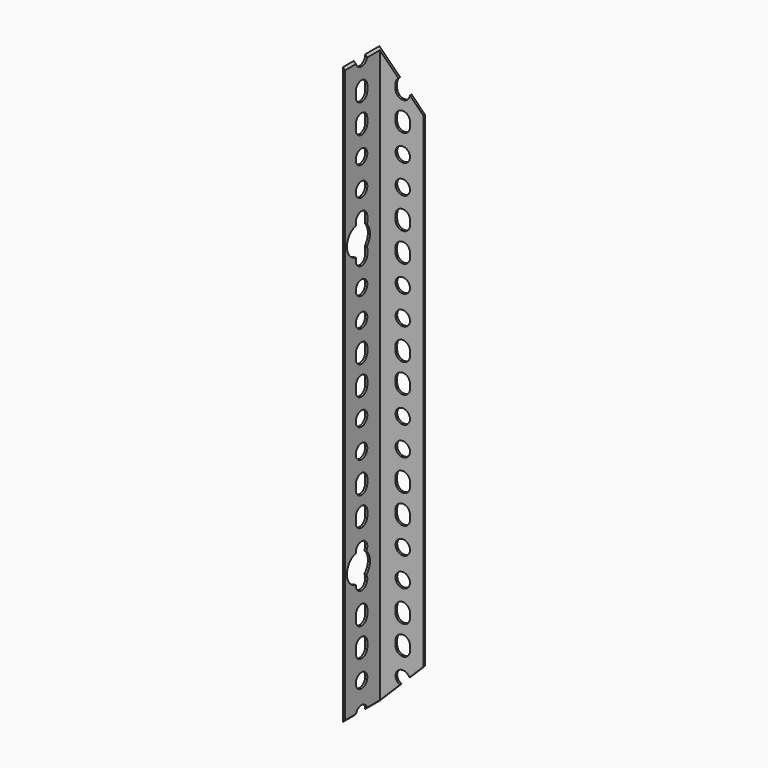
from build123d import *

# Parameters (mm, degrees)
F2_DEPTH  = 381
F3_R      = 4.7625
F5_DEPTH  = 1.3726
F4_R      = 4.7625
F6_DEPTH  = 1.3726
F8_DEPTH  = 30.1254
F10_DEPTH = 30.1254


# Not quite as in the source:
# - a variable given as a bare number and used for a length is read in inches; the dataset says mm whatever the document's units were


with BuildPart() as f2:
    # F1 (on Top) → F2 (new body)
    with BuildSketch(Plane.XY):
        Polygon((-1.3716, 1.3716), (-1.3716, -28.7528), (0, -28.7528), (0, 0), (28.7528, 0), (28.7528, 1.3716), align=None)
    extrude(amount=F2_DEPTH)

    # F3 (on face) → F5 (cut, through all)
    with BuildSketch(Plane.XZ):
        with Locations((15.1384, 19.05)):
            Circle(F3_R)
        with Locations((15.1384, 0)):
            Circle(F3_R)
        with BuildLine():
            Line((19.9009, 36.5125), (19.9009, 39.6875))
            ThreePointArc((19.9009, 39.6875), (15.1384, 44.45), (10.3759, 39.6875))
            Line((10.3759, 39.6875), (10.3759, 36.5125))
            ThreePointArc((10.3759, 36.5125), (15.1384, 31.75), (19.9009, 36.5125))
        make_face()
        with BuildLine():
            Line((19.9009, 55.5625), (19.9009, 58.7375))
            ThreePointArc((19.9009, 58.7375), (15.1384, 63.5), (10.3759, 58.7375))
            Line((10.3759, 58.7375), (10.3759, 55.5625))
            ThreePointArc((10.3759, 55.5625), (15.1384, 50.8), (19.9009, 55.5625))
        make_face()
        with BuildLine():
            Line((19.9009, 131.7625), (19.9009, 134.9375))
            ThreePointArc((19.9009, 134.9375), (15.1384, 139.7), (10.3759, 134.9375))
            Line((10.3759, 134.9375), (10.3759, 131.7625))
            ThreePointArc((10.3759, 131.7625), (15.1384, 127), (19.9009, 131.7625))
        make_face()
        with Locations((15.1384, 95.25)):
            Circle(F3_R)
        with Locations((15.1384, 76.2)):
            Circle(F3_R)
        with BuildLine():
            Line((19.9009, 112.7125), (19.9009, 115.8875))
            ThreePointArc((19.9009, 115.8875), (15.1384, 120.65), (10.3759, 115.8875))
            Line((10.3759, 115.8875), (10.3759, 112.7125))
            ThreePointArc((10.3759, 112.7125), (15.1384, 107.95), (19.9009, 112.7125))
        make_face()
        with BuildLine():
            Line((19.9009, 207.9625), (19.9009, 211.1375))
            ThreePointArc((19.9009, 211.1375), (15.1384, 215.9), (10.3759, 211.1375))
            Line((10.3759, 211.1375), (10.3759, 207.9625))
            ThreePointArc((10.3759, 207.9625), (15.1384, 203.2), (19.9009, 207.9625))
        make_face()
        with Locations((15.1384, 171.45)):
            Circle(F3_R)
        with Locations((15.1384, 152.4)):
            Circle(F3_R)
        with BuildLine():
            Line((19.9009, 188.9125), (19.9009, 192.0875))
            ThreePointArc((19.9009, 192.0875), (15.1384, 196.85), (10.3759, 192.0875))
            Line((10.3759, 192.0875), (10.3759, 188.9125))
            ThreePointArc((10.3759, 188.9125), (15.1384, 184.15), (19.9009, 188.9125))
        make_face()
        with BuildLine():
            Line((19.9009, 284.1625), (19.9009, 287.3375))
            ThreePointArc((19.9009, 287.3375), (15.1384, 292.1), (10.3759, 287.3375))
            Line((10.3759, 287.3375), (10.3759, 284.1625))
            ThreePointArc((10.3759, 284.1625), (15.1384, 279.4), (19.9009, 284.1625))
        make_face()
        with Locations((15.1384, 247.65)):
            Circle(F3_R)
        with Locations((15.1384, 228.6)):
            Circle(F3_R)
        with BuildLine():
            Line((19.9009, 265.1125), (19.9009, 268.2875))
            ThreePointArc((19.9009, 268.2875), (15.1384, 273.05), (10.3759, 268.2875))
            Line((10.3759, 268.2875), (10.3759, 265.1125))
            ThreePointArc((10.3759, 265.1125), (15.1384, 260.35), (19.9009, 265.1125))
        make_face()
        with BuildLine():
            Line((19.9009, 360.3625), (19.9009, 363.5375))
            ThreePointArc((19.9009, 363.5375), (15.1384, 368.3), (10.3759, 363.5375))
            Line((10.3759, 363.5375), (10.3759, 360.3625))
            ThreePointArc((10.3759, 360.3625), (15.1384, 355.6), (19.9009, 360.3625))
        make_face()
        with Locations((15.1384, 323.85)):
            Circle(F3_R)
        with Locations((15.1384, 304.8)):
            Circle(F3_R)
        with BuildLine():
            Line((19.9009, 341.3125), (19.9009, 344.4875))
            ThreePointArc((19.9009, 344.4875), (15.1384, 349.25), (10.3759, 344.4875))
            Line((10.3759, 344.4875), (10.3759, 341.3125))
            ThreePointArc((10.3759, 341.3125), (15.1384, 336.55), (19.9009, 341.3125))
        make_face()
        with BuildLine():
            Line((19.9009, 436.5625), (19.9009, 439.7375))
            ThreePointArc((19.9009, 439.7375), (15.1384, 444.5), (10.3759, 439.7375))
            Line((10.3759, 439.7375), (10.3759, 436.5625))
            ThreePointArc((10.3759, 436.5625), (15.1384, 431.8), (19.9009, 436.5625))
        make_face()
        with Locations((15.1384, 400.05)):
            Circle(F3_R)
        with Locations((15.1384, 381)):
            Circle(F3_R)
        with BuildLine():
            Line((19.9009, 417.5125), (19.9009, 420.6875))
            ThreePointArc((19.9009, 420.6875), (15.1384, 425.45), (10.3759, 420.6875))
            Line((10.3759, 420.6875), (10.3759, 417.5125))
            ThreePointArc((10.3759, 417.5125), (15.1384, 412.75), (19.9009, 417.5125))
        make_face()
        with BuildLine():
            Line((19.9009, 512.7625), (19.9009, 515.9375))
            ThreePointArc((19.9009, 515.9375), (15.1384, 520.7), (10.3759, 515.9375))
            Line((10.3759, 515.9375), (10.3759, 512.7625))
            ThreePointArc((10.3759, 512.7625), (15.1384, 508), (19.9009, 512.7625))
        make_face()
        with Locations((15.1384, 476.25)):
            Circle(F3_R)
        with Locations((15.1384, 457.2)):
            Circle(F3_R)
        with BuildLine():
            Line((19.9009, 493.7125), (19.9009, 496.8875))
            ThreePointArc((19.9009, 496.8875), (15.1384, 501.65), (10.3759, 496.8875))
            Line((10.3759, 496.8875), (10.3759, 493.7125))
            ThreePointArc((10.3759, 493.7125), (15.1384, 488.95), (19.9009, 493.7125))
        make_face()
        with BuildLine():
            Line((19.9009, 588.9625), (19.9009, 592.1375))
            ThreePointArc((19.9009, 592.1375), (15.1384, 596.9), (10.3759, 592.1375))
            Line((10.3759, 592.1375), (10.3759, 588.9625))
            ThreePointArc((10.3759, 588.9625), (15.1384, 584.2), (19.9009, 588.9625))
        make_face()
        with Locations((15.1384, 552.45)):
            Circle(F3_R)
        with Locations((15.1384, 533.4)):
            Circle(F3_R)
        with BuildLine():
            Line((19.9009, 569.9125), (19.9009, 573.0875))
            ThreePointArc((19.9009, 573.0875), (15.1384, 577.85), (10.3759, 573.0875))
            Line((10.3759, 573.0875), (10.3759, 569.9125))
            ThreePointArc((10.3759, 569.9125), (15.1384, 565.15), (19.9009, 569.9125))
        make_face()
        with BuildLine():
            Line((19.9009, 665.1625), (19.9009, 668.3375))
            ThreePointArc((19.9009, 668.3375), (15.1384, 673.1), (10.3759, 668.3375))
            Line((10.3759, 668.3375), (10.3759, 665.1625))
            ThreePointArc((10.3759, 665.1625), (15.1384, 660.4), (19.9009, 665.1625))
        make_face()
        with Locations((15.1384, 628.65)):
            Circle(F3_R)
        with Locations((15.1384, 609.6)):
            Circle(F3_R)
        with BuildLine():
            Line((19.9009, 646.1125), (19.9009, 649.2875))
            ThreePointArc((19.9009, 649.2875), (15.1384, 654.05), (10.3759, 649.2875))
            Line((10.3759, 649.2875), (10.3759, 646.1125))
            ThreePointArc((10.3759, 646.1125), (15.1384, 641.35), (19.9009, 646.1125))
        make_face()
        with BuildLine():
            Line((19.9009, 741.3625), (19.9009, 744.5375))
            ThreePointArc((19.9009, 744.5375), (15.1384, 749.3), (10.3759, 744.5375))
            Line((10.3759, 744.5375), (10.3759, 741.3625))
            ThreePointArc((10.3759, 741.3625), (15.1384, 736.6), (19.9009, 741.3625))
        make_face()
        with Locations((15.1384, 704.85)):
            Circle(F3_R)
        with Locations((15.1384, 685.8)):
            Circle(F3_R)
        with BuildLine():
            Line((19.9009, 722.3125), (19.9009, 725.4875))
            ThreePointArc((19.9009, 725.4875), (15.1384, 730.25), (10.3759, 725.4875))
            Line((10.3759, 725.4875), (10.3759, 722.3125))
            ThreePointArc((10.3759, 722.3125), (15.1384, 717.55), (19.9009, 722.3125))
        make_face()
        with BuildLine():
            Line((19.9009, 817.5625), (19.9009, 820.7375))
            ThreePointArc((19.9009, 820.7375), (15.1384, 825.5), (10.3759, 820.7375))
            Line((10.3759, 820.7375), (10.3759, 817.5625))
            ThreePointArc((10.3759, 817.5625), (15.1384, 812.8), (19.9009, 817.5625))
        make_face()
        with Locations((15.1384, 781.05)):
            Circle(F3_R)
        with Locations((15.1384, 762)):
            Circle(F3_R)
        with BuildLine():
            Line((19.9009, 798.5125), (19.9009, 801.6875))
            ThreePointArc((19.9009, 801.6875), (15.1384, 806.45), (10.3759, 801.6875))
            Line((10.3759, 801.6875), (10.3759, 798.5125))
            ThreePointArc((10.3759, 798.5125), (15.1384, 793.75), (19.9009, 798.5125))
        make_face()
        with BuildLine():
            Line((19.9009, 893.7625), (19.9009, 896.9375))
            ThreePointArc((19.9009, 896.9375), (15.1384, 901.7), (10.3759, 896.9375))
            Line((10.3759, 896.9375), (10.3759, 893.7625))
            ThreePointArc((10.3759, 893.7625), (15.1384, 889), (19.9009, 893.7625))
        make_face()
        with Locations((15.1384, 857.25)):
            Circle(F3_R)
        with Locations((15.1384, 838.2)):
            Circle(F3_R)
        with BuildLine():
            Line((19.9009, 874.7125), (19.9009, 877.8875))
            ThreePointArc((19.9009, 877.8875), (15.1384, 882.65), (10.3759, 877.8875))
            Line((10.3759, 877.8875), (10.3759, 874.7125))
            ThreePointArc((10.3759, 874.7125), (15.1384, 869.95), (19.9009, 874.7125))
        make_face()
        with BuildLine():
            Line((19.9009, 969.9625), (19.9009, 973.1375))
            ThreePointArc((19.9009, 973.1375), (15.1384, 977.9), (10.3759, 973.1375))
            Line((10.3759, 973.1375), (10.3759, 969.9625))
            ThreePointArc((10.3759, 969.9625), (15.1384, 965.2), (19.9009, 969.9625))
        make_face()
        with Locations((15.1384, 933.45)):
            Circle(F3_R)
        with Locations((15.1384, 914.4)):
            Circle(F3_R)
        with BuildLine():
            Line((19.9009, 950.9125), (19.9009, 954.0875))
            ThreePointArc((19.9009, 954.0875), (15.1384, 958.85), (10.3759, 954.0875))
            Line((10.3759, 954.0875), (10.3759, 950.9125))
            ThreePointArc((10.3759, 950.9125), (15.1384, 946.15), (19.9009, 950.9125))
        make_face()
        with BuildLine():
            Line((19.9009, 1046.1625), (19.9009, 1049.3375))
            ThreePointArc((19.9009, 1049.3375), (15.1384, 1054.1), (10.3759, 1049.3375))
            Line((10.3759, 1049.3375), (10.3759, 1046.1625))
            ThreePointArc((10.3759, 1046.1625), (15.1384, 1041.4), (19.9009, 1046.1625))
        make_face()
        with Locations((15.1384, 1009.65)):
            Circle(F3_R)
        with Locations((15.1384, 990.6)):
            Circle(F3_R)
        with BuildLine():
            Line((19.9009, 1027.1125), (19.9009, 1030.2875))
            ThreePointArc((19.9009, 1030.2875), (15.1384, 1035.05), (10.3759, 1030.2875))
            Line((10.3759, 1030.2875), (10.3759, 1027.1125))
            ThreePointArc((10.3759, 1027.1125), (15.1384, 1022.35), (19.9009, 1027.1125))
        make_face()
        with BuildLine():
            Line((19.9009, 1122.3625), (19.9009, 1125.5375))
            ThreePointArc((19.9009, 1125.5375), (15.1384, 1130.3), (10.3759, 1125.5375))
            Line((10.3759, 1125.5375), (10.3759, 1122.3625))
            ThreePointArc((10.3759, 1122.3625), (15.1384, 1117.6), (19.9009, 1122.3625))
        make_face()
        with Locations((15.1384, 1085.85)):
            Circle(F3_R)
        with Locations((15.1384, 1066.8)):
            Circle(F3_R)
        with BuildLine():
            Line((19.9009, 1103.3125), (19.9009, 1106.4875))
            ThreePointArc((19.9009, 1106.4875), (15.1384, 1111.25), (10.3759, 1106.4875))
            Line((10.3759, 1106.4875), (10.3759, 1103.3125))
            ThreePointArc((10.3759, 1103.3125), (15.1384, 1098.55), (19.9009, 1103.3125))
        make_face()
        with BuildLine():
            Line((19.9009, 1198.5625), (19.9009, 1201.7375))
            ThreePointArc((19.9009, 1201.7375), (15.1384, 1206.5), (10.3759, 1201.7375))
            Line((10.3759, 1201.7375), (10.3759, 1198.5625))
            ThreePointArc((10.3759, 1198.5625), (15.1384, 1193.8), (19.9009, 1198.5625))
        make_face()
        with Locations((15.1384, 1162.05)):
            Circle(F3_R)
        with Locations((15.1384, 1143)):
            Circle(F3_R)
        with BuildLine():
            Line((19.9009, 1179.5125), (19.9009, 1182.6875))
            ThreePointArc((19.9009, 1182.6875), (15.1384, 1187.45), (10.3759, 1182.6875))
            Line((10.3759, 1182.6875), (10.3759, 1179.5125))
            ThreePointArc((10.3759, 1179.5125), (15.1384, 1174.75), (19.9009, 1179.5125))
        make_face()
        with BuildLine():
            Line((19.9009, 1274.7625), (19.9009, 1277.9375))
            ThreePointArc((19.9009, 1277.9375), (15.1384, 1282.7), (10.3759, 1277.9375))
            Line((10.3759, 1277.9375), (10.3759, 1274.7625))
            ThreePointArc((10.3759, 1274.7625), (15.1384, 1270), (19.9009, 1274.7625))
        make_face()
        with Locations((15.1384, 1238.25)):
            Circle(F3_R)
        with Locations((15.1384, 1219.2)):
            Circle(F3_R)
        with BuildLine():
            Line((19.9009, 1255.7125), (19.9009, 1258.8875))
            ThreePointArc((19.9009, 1258.8875), (15.1384, 1263.65), (10.3759, 1258.8875))
            Line((10.3759, 1258.8875), (10.3759, 1255.7125))
            ThreePointArc((10.3759, 1255.7125), (15.1384, 1250.95), (19.9009, 1255.7125))
        make_face()
        with BuildLine():
            Line((19.9009, 1350.9625), (19.9009, 1354.1375))
            ThreePointArc((19.9009, 1354.1375), (15.1384, 1358.9), (10.3759, 1354.1375))
            Line((10.3759, 1354.1375), (10.3759, 1350.9625))
            ThreePointArc((10.3759, 1350.9625), (15.1384, 1346.2), (19.9009, 1350.9625))
        make_face()
        with Locations((15.1384, 1314.45)):
            Circle(F3_R)
        with Locations((15.1384, 1295.4)):
            Circle(F3_R)
        with BuildLine():
            Line((19.9009, 1331.9125), (19.9009, 1335.0875))
            ThreePointArc((19.9009, 1335.0875), (15.1384, 1339.85), (10.3759, 1335.0875))
            Line((10.3759, 1335.0875), (10.3759, 1331.9125))
            ThreePointArc((10.3759, 1331.9125), (15.1384, 1327.15), (19.9009, 1331.9125))
        make_face()
        with BuildLine():
            Line((19.9009, 1427.1625), (19.9009, 1430.3375))
            ThreePointArc((19.9009, 1430.3375), (15.1384, 1435.1), (10.3759, 1430.3375))
            Line((10.3759, 1430.3375), (10.3759, 1427.1625))
            ThreePointArc((10.3759, 1427.1625), (15.1384, 1422.4), (19.9009, 1427.1625))
        make_face()
        with Locations((15.1384, 1390.65)):
            Circle(F3_R)
        with Locations((15.1384, 1371.6)):
            Circle(F3_R)
        with BuildLine():
            Line((19.9009, 1408.1125), (19.9009, 1411.2875))
            ThreePointArc((19.9009, 1411.2875), (15.1384, 1416.05), (10.3759, 1411.2875))
            Line((10.3759, 1411.2875), (10.3759, 1408.1125))
            ThreePointArc((10.3759, 1408.1125), (15.1384, 1403.35), (19.9009, 1408.1125))
        make_face()
        with BuildLine():
            Line((19.9009, 1503.3625), (19.9009, 1506.5375))
            ThreePointArc((19.9009, 1506.5375), (15.1384, 1511.3), (10.3759, 1506.5375))
            Line((10.3759, 1506.5375), (10.3759, 1503.3625))
            ThreePointArc((10.3759, 1503.3625), (15.1384, 1498.6), (19.9009, 1503.3625))
        make_face()
        with Locations((15.1384, 1466.85)):
            Circle(F3_R)
        with Locations((15.1384, 1447.8)):
            Circle(F3_R)
        with BuildLine():
            Line((19.9009, 1484.3125), (19.9009, 1487.4875))
            ThreePointArc((19.9009, 1487.4875), (15.1384, 1492.25), (10.3759, 1487.4875))
            Line((10.3759, 1487.4875), (10.3759, 1484.3125))
            ThreePointArc((10.3759, 1484.3125), (15.1384, 1479.55), (19.9009, 1484.3125))
        make_face()
        with BuildLine():
            Line((19.9009, 1579.5625), (19.9009, 1582.7375))
            ThreePointArc((19.9009, 1582.7375), (15.1384, 1587.5), (10.3759, 1582.7375))
            Line((10.3759, 1582.7375), (10.3759, 1579.5625))
            ThreePointArc((10.3759, 1579.5625), (15.1384, 1574.8), (19.9009, 1579.5625))
        make_face()
        with Locations((15.1384, 1543.05)):
            Circle(F3_R)
        with Locations((15.1384, 1524)):
            Circle(F3_R)
        with BuildLine():
            Line((19.9009, 1560.5125), (19.9009, 1563.6875))
            ThreePointArc((19.9009, 1563.6875), (15.1384, 1568.45), (10.3759, 1563.6875))
            Line((10.3759, 1563.6875), (10.3759, 1560.5125))
            ThreePointArc((10.3759, 1560.5125), (15.1384, 1555.75), (19.9009, 1560.5125))
        make_face()
        with BuildLine():
            Line((19.9009, 1655.7625), (19.9009, 1658.9375))
            ThreePointArc((19.9009, 1658.9375), (15.1384, 1663.7), (10.3759, 1658.9375))
            Line((10.3759, 1658.9375), (10.3759, 1655.7625))
            ThreePointArc((10.3759, 1655.7625), (15.1384, 1651), (19.9009, 1655.7625))
        make_face()
        with Locations((15.1384, 1619.25)):
            Circle(F3_R)
        with Locations((15.1384, 1600.2)):
            Circle(F3_R)
        with BuildLine():
            Line((19.9009, 1636.7125), (19.9009, 1639.8875))
            ThreePointArc((19.9009, 1639.8875), (15.1384, 1644.65), (10.3759, 1639.8875))
            Line((10.3759, 1639.8875), (10.3759, 1636.7125))
            ThreePointArc((10.3759, 1636.7125), (15.1384, 1631.95), (19.9009, 1636.7125))
        make_face()
        with BuildLine():
            Line((19.9009, 1731.9625), (19.9009, 1735.1375))
            ThreePointArc((19.9009, 1735.1375), (15.1384, 1739.9), (10.3759, 1735.1375))
            Line((10.3759, 1735.1375), (10.3759, 1731.9625))
            ThreePointArc((10.3759, 1731.9625), (15.1384, 1727.2), (19.9009, 1731.9625))
        make_face()
        with Locations((15.1384, 1695.45)):
            Circle(F3_R)
        with Locations((15.1384, 1676.4)):
            Circle(F3_R)
        with BuildLine():
            Line((19.9009, 1712.9125), (19.9009, 1716.0875))
            ThreePointArc((19.9009, 1716.0875), (15.1384, 1720.85), (10.3759, 1716.0875))
            Line((10.3759, 1716.0875), (10.3759, 1712.9125))
            ThreePointArc((10.3759, 1712.9125), (15.1384, 1708.15), (19.9009, 1712.9125))
        make_face()
        with BuildLine():
            Line((19.9009, 1808.1625), (19.9009, 1811.3375))
            ThreePointArc((19.9009, 1811.3375), (15.1384, 1816.1), (10.3759, 1811.3375))
            Line((10.3759, 1811.3375), (10.3759, 1808.1625))
            ThreePointArc((10.3759, 1808.1625), (15.1384, 1803.4), (19.9009, 1808.1625))
        make_face()
        with Locations((15.1384, 1771.65)):
            Circle(F3_R)
        with Locations((15.1384, 1752.6)):
            Circle(F3_R)
        with BuildLine():
            Line((19.9009, 1789.1125), (19.9009, 1792.2875))
            ThreePointArc((19.9009, 1792.2875), (15.1384, 1797.05), (10.3759, 1792.2875))
            Line((10.3759, 1792.2875), (10.3759, 1789.1125))
            ThreePointArc((10.3759, 1789.1125), (15.1384, 1784.35), (19.9009, 1789.1125))
        make_face()
    extrude(amount=-F5_DEPTH, mode=Mode.SUBTRACT)

    # F4 (on face) → F6 (cut, through all)
    with BuildSketch(Plane.YZ):
        with Locations((-15.1384, 19.05)):
            Circle(F4_R)
        with Locations((-15.1384, 0)):
            Circle(F4_R)
        with BuildLine():
            Line((-10.3759, 36.5125), (-10.3759, 39.6875))
            ThreePointArc((-10.3759, 39.6875), (-15.1384, 44.45), (-19.9009, 39.6875))
            Line((-19.9009, 39.6875), (-19.9009, 36.5125))
            ThreePointArc((-19.9009, 36.5125), (-15.1384, 31.75), (-10.3759, 36.5125))
        make_face()
        with BuildLine():
            Line((-10.3759, 55.5625), (-10.3759, 58.7375))
            ThreePointArc((-10.3759, 58.7375), (-15.1384, 63.5), (-19.9009, 58.7375))
            Line((-19.9009, 58.7375), (-19.9009, 55.5625))
            ThreePointArc((-19.9009, 55.5625), (-15.1384, 50.8), (-10.3759, 55.5625))
        make_face()
        with BuildLine():
            Line((-10.3759, 131.7625), (-10.3759, 134.9375))
            ThreePointArc((-10.3759, 134.9375), (-15.1384, 139.7), (-19.9009, 134.9375))
            Line((-19.9009, 134.9375), (-19.9009, 131.7625))
            ThreePointArc((-19.9009, 131.7625), (-15.1384, 127), (-10.3759, 131.7625))
        make_face()
        with Locations((-15.1384, 95.25)):
            Circle(F4_R)
        with Locations((-15.1384, 76.2)):
            Circle(F4_R)
        with BuildLine():
            Line((-10.3759, 112.7125), (-10.3759, 115.8875))
            ThreePointArc((-10.3759, 115.8875), (-15.1384, 120.65), (-19.9009, 115.8875))
            Line((-19.9009, 115.8875), (-19.9009, 112.7125))
            ThreePointArc((-19.9009, 112.7125), (-15.1384, 107.95), (-10.3759, 112.7125))
        make_face()
        with BuildLine():
            Line((-10.3759, 207.9625), (-10.3759, 211.1375))
            ThreePointArc((-10.3759, 211.1375), (-15.1384, 215.9), (-19.9009, 211.1375))
            Line((-19.9009, 211.1375), (-19.9009, 207.9625))
            ThreePointArc((-19.9009, 207.9625), (-15.1384, 203.2), (-10.3759, 207.9625))
        make_face()
        with Locations((-15.1384, 171.45)):
            Circle(F4_R)
        with Locations((-15.1384, 152.4)):
            Circle(F4_R)
        with BuildLine():
            Line((-10.3759, 188.9125), (-10.3759, 192.0875))
            ThreePointArc((-10.3759, 192.0875), (-15.1384, 196.85), (-19.9009, 192.0875))
            Line((-19.9009, 192.0875), (-19.9009, 188.9125))
            ThreePointArc((-19.9009, 188.9125), (-15.1384, 184.15), (-10.3759, 188.9125))
        make_face()
        with BuildLine():
            Line((-10.3759, 284.1625), (-10.3759, 287.3375))
            ThreePointArc((-10.3759, 287.3375), (-15.1384, 292.1), (-19.9009, 287.3375))
            Line((-19.9009, 287.3375), (-19.9009, 284.1625))
            ThreePointArc((-19.9009, 284.1625), (-15.1384, 279.4), (-10.3759, 284.1625))
        make_face()
        with Locations((-15.1384, 247.65)):
            Circle(F4_R)
        with Locations((-15.1384, 228.6)):
            Circle(F4_R)
        with BuildLine():
            Line((-10.3759, 265.1125), (-10.3759, 268.2875))
            ThreePointArc((-10.3759, 268.2875), (-15.1384, 273.05), (-19.9009, 268.2875))
            Line((-19.9009, 268.2875), (-19.9009, 265.1125))
            ThreePointArc((-19.9009, 265.1125), (-15.1384, 260.35), (-10.3759, 265.1125))
        make_face()
        with BuildLine():
            Line((-10.3759, 360.3625), (-10.3759, 363.5375))
            ThreePointArc((-10.3759, 363.5375), (-15.1384, 368.3), (-19.9009, 363.5375))
            Line((-19.9009, 363.5375), (-19.9009, 360.3625))
            ThreePointArc((-19.9009, 360.3625), (-15.1384, 355.6), (-10.3759, 360.3625))
        make_face()
        with Locations((-15.1384, 323.85)):
            Circle(F4_R)
        with Locations((-15.1384, 304.8)):
            Circle(F4_R)
        with BuildLine():
            Line((-10.3759, 341.3125), (-10.3759, 344.4875))
            ThreePointArc((-10.3759, 344.4875), (-15.1384, 349.25), (-19.9009, 344.4875))
            Line((-19.9009, 344.4875), (-19.9009, 341.3125))
            ThreePointArc((-19.9009, 341.3125), (-15.1384, 336.55), (-10.3759, 341.3125))
        make_face()
        with BuildLine():
            Line((-10.3759, 436.5625), (-10.3759, 439.7375))
            ThreePointArc((-10.3759, 439.7375), (-15.1384, 444.5), (-19.9009, 439.7375))
            Line((-19.9009, 439.7375), (-19.9009, 436.5625))
            ThreePointArc((-19.9009, 436.5625), (-15.1384, 431.8), (-10.3759, 436.5625))
        make_face()
        with Locations((-15.1384, 400.05)):
            Circle(F4_R)
        with Locations((-15.1384, 381)):
            Circle(F4_R)
        with BuildLine():
            Line((-10.3759, 417.5125), (-10.3759, 420.6875))
            ThreePointArc((-10.3759, 420.6875), (-15.1384, 425.45), (-19.9009, 420.6875))
            Line((-19.9009, 420.6875), (-19.9009, 417.5125))
            ThreePointArc((-19.9009, 417.5125), (-15.1384, 412.75), (-10.3759, 417.5125))
        make_face()
        with BuildLine():
            Line((-10.3759, 512.7625), (-10.3759, 515.9375))
            ThreePointArc((-10.3759, 515.9375), (-15.1384, 520.7), (-19.9009, 515.9375))
            Line((-19.9009, 515.9375), (-19.9009, 512.7625))
            ThreePointArc((-19.9009, 512.7625), (-15.1384, 508), (-10.3759, 512.7625))
        make_face()
        with Locations((-15.1384, 476.25)):
            Circle(F4_R)
        with Locations((-15.1384, 457.2)):
            Circle(F4_R)
        with BuildLine():
            Line((-10.3759, 493.7125), (-10.3759, 496.8875))
            ThreePointArc((-10.3759, 496.8875), (-15.1384, 501.65), (-19.9009, 496.8875))
            Line((-19.9009, 496.8875), (-19.9009, 493.7125))
            ThreePointArc((-19.9009, 493.7125), (-15.1384, 488.95), (-10.3759, 493.7125))
        make_face()
        with BuildLine():
            Line((-10.3759, 588.9625), (-10.3759, 592.1375))
            ThreePointArc((-10.3759, 592.1375), (-15.1384, 596.9), (-19.9009, 592.1375))
            Line((-19.9009, 592.1375), (-19.9009, 588.9625))
            ThreePointArc((-19.9009, 588.9625), (-15.1384, 584.2), (-10.3759, 588.9625))
        make_face()
        with Locations((-15.1384, 552.45)):
            Circle(F4_R)
        with Locations((-15.1384, 533.4)):
            Circle(F4_R)
        with BuildLine():
            Line((-10.3759, 569.9125), (-10.3759, 573.0875))
            ThreePointArc((-10.3759, 573.0875), (-15.1384, 577.85), (-19.9009, 573.0875))
            Line((-19.9009, 573.0875), (-19.9009, 569.9125))
            ThreePointArc((-19.9009, 569.9125), (-15.1384, 565.15), (-10.3759, 569.9125))
        make_face()
        with BuildLine():
            Line((-10.3759, 665.1625), (-10.3759, 668.3375))
            ThreePointArc((-10.3759, 668.3375), (-15.1384, 673.1), (-19.9009, 668.3375))
            Line((-19.9009, 668.3375), (-19.9009, 665.1625))
            ThreePointArc((-19.9009, 665.1625), (-15.1384, 660.4), (-10.3759, 665.1625))
        make_face()
        with Locations((-15.1384, 628.65)):
            Circle(F4_R)
        with Locations((-15.1384, 609.6)):
            Circle(F4_R)
        with BuildLine():
            Line((-10.3759, 646.1125), (-10.3759, 649.2875))
            ThreePointArc((-10.3759, 649.2875), (-15.1384, 654.05), (-19.9009, 649.2875))
            Line((-19.9009, 649.2875), (-19.9009, 646.1125))
            ThreePointArc((-19.9009, 646.1125), (-15.1384, 641.35), (-10.3759, 646.1125))
        make_face()
        with BuildLine():
            Line((-10.3759, 741.3625), (-10.3759, 744.5375))
            ThreePointArc((-10.3759, 744.5375), (-15.1384, 749.3), (-19.9009, 744.5375))
            Line((-19.9009, 744.5375), (-19.9009, 741.3625))
            ThreePointArc((-19.9009, 741.3625), (-15.1384, 736.6), (-10.3759, 741.3625))
        make_face()
        with Locations((-15.1384, 704.85)):
            Circle(F4_R)
        with Locations((-15.1384, 685.8)):
            Circle(F4_R)
        with BuildLine():
            Line((-10.3759, 722.3125), (-10.3759, 725.4875))
            ThreePointArc((-10.3759, 725.4875), (-15.1384, 730.25), (-19.9009, 725.4875))
            Line((-19.9009, 725.4875), (-19.9009, 722.3125))
            ThreePointArc((-19.9009, 722.3125), (-15.1384, 717.55), (-10.3759, 722.3125))
        make_face()
        with BuildLine():
            Line((-10.3759, 817.5625), (-10.3759, 820.7375))
            ThreePointArc((-10.3759, 820.7375), (-15.1384, 825.5), (-19.9009, 820.7375))
            Line((-19.9009, 820.7375), (-19.9009, 817.5625))
            ThreePointArc((-19.9009, 817.5625), (-15.1384, 812.8), (-10.3759, 817.5625))
        make_face()
        with Locations((-15.1384, 781.05)):
            Circle(F4_R)
        with Locations((-15.1384, 762)):
            Circle(F4_R)
        with BuildLine():
            Line((-10.3759, 798.5125), (-10.3759, 801.6875))
            ThreePointArc((-10.3759, 801.6875), (-15.1384, 806.45), (-19.9009, 801.6875))
            Line((-19.9009, 801.6875), (-19.9009, 798.5125))
            ThreePointArc((-19.9009, 798.5125), (-15.1384, 793.75), (-10.3759, 798.5125))
        make_face()
        with BuildLine():
            Line((-10.3759, 893.7625), (-10.3759, 896.9375))
            ThreePointArc((-10.3759, 896.9375), (-15.1384, 901.7), (-19.9009, 896.9375))
            Line((-19.9009, 896.9375), (-19.9009, 893.7625))
            ThreePointArc((-19.9009, 893.7625), (-15.1384, 889), (-10.3759, 893.7625))
        make_face()
        with Locations((-15.1384, 857.25)):
            Circle(F4_R)
        with Locations((-15.1384, 838.2)):
            Circle(F4_R)
        with BuildLine():
            Line((-10.3759, 874.7125), (-10.3759, 877.8875))
            ThreePointArc((-10.3759, 877.8875), (-15.1384, 882.65), (-19.9009, 877.8875))
            Line((-19.9009, 877.8875), (-19.9009, 874.7125))
            ThreePointArc((-19.9009, 874.7125), (-15.1384, 869.95), (-10.3759, 874.7125))
        make_face()
        with BuildLine():
            Line((-10.3759, 969.9625), (-10.3759, 973.1375))
            ThreePointArc((-10.3759, 973.1375), (-15.1384, 977.9), (-19.9009, 973.1375))
            Line((-19.9009, 973.1375), (-19.9009, 969.9625))
            ThreePointArc((-19.9009, 969.9625), (-15.1384, 965.2), (-10.3759, 969.9625))
        make_face()
        with Locations((-15.1384, 933.45)):
            Circle(F4_R)
        with Locations((-15.1384, 914.4)):
            Circle(F4_R)
        with BuildLine():
            Line((-10.3759, 950.9125), (-10.3759, 954.0875))
            ThreePointArc((-10.3759, 954.0875), (-15.1384, 958.85), (-19.9009, 954.0875))
            Line((-19.9009, 954.0875), (-19.9009, 950.9125))
            ThreePointArc((-19.9009, 950.9125), (-15.1384, 946.15), (-10.3759, 950.9125))
        make_face()
        with BuildLine():
            Line((-10.3759, 1046.1625), (-10.3759, 1049.3375))
            ThreePointArc((-10.3759, 1049.3375), (-15.1384, 1054.1), (-19.9009, 1049.3375))
            Line((-19.9009, 1049.3375), (-19.9009, 1046.1625))
            ThreePointArc((-19.9009, 1046.1625), (-15.1384, 1041.4), (-10.3759, 1046.1625))
        make_face()
        with Locations((-15.1384, 1009.65)):
            Circle(F4_R)
        with Locations((-15.1384, 990.6)):
            Circle(F4_R)
        with BuildLine():
            Line((-10.3759, 1027.1125), (-10.3759, 1030.2875))
            ThreePointArc((-10.3759, 1030.2875), (-15.1384, 1035.05), (-19.9009, 1030.2875))
            Line((-19.9009, 1030.2875), (-19.9009, 1027.1125))
            ThreePointArc((-19.9009, 1027.1125), (-15.1384, 1022.35), (-10.3759, 1027.1125))
        make_face()
        with BuildLine():
            Line((-10.3759, 1122.3625), (-10.3759, 1125.5375))
            ThreePointArc((-10.3759, 1125.5375), (-15.1384, 1130.3), (-19.9009, 1125.5375))
            Line((-19.9009, 1125.5375), (-19.9009, 1122.3625))
            ThreePointArc((-19.9009, 1122.3625), (-15.1384, 1117.6), (-10.3759, 1122.3625))
        make_face()
        with Locations((-15.1384, 1085.85)):
            Circle(F4_R)
        with Locations((-15.1384, 1066.8)):
            Circle(F4_R)
        with BuildLine():
            Line((-10.3759, 1103.3125), (-10.3759, 1106.4875))
            ThreePointArc((-10.3759, 1106.4875), (-15.1384, 1111.25), (-19.9009, 1106.4875))
            Line((-19.9009, 1106.4875), (-19.9009, 1103.3125))
            ThreePointArc((-19.9009, 1103.3125), (-15.1384, 1098.55), (-10.3759, 1103.3125))
        make_face()
        with BuildLine():
            Line((-10.3759, 1198.5625), (-10.3759, 1201.7375))
            ThreePointArc((-10.3759, 1201.7375), (-15.1384, 1206.5), (-19.9009, 1201.7375))
            Line((-19.9009, 1201.7375), (-19.9009, 1198.5625))
            ThreePointArc((-19.9009, 1198.5625), (-15.1384, 1193.8), (-10.3759, 1198.5625))
        make_face()
        with Locations((-15.1384, 1162.05)):
            Circle(F4_R)
        with Locations((-15.1384, 1143)):
            Circle(F4_R)
        with BuildLine():
            Line((-10.3759, 1179.5125), (-10.3759, 1182.6875))
            ThreePointArc((-10.3759, 1182.6875), (-15.1384, 1187.45), (-19.9009, 1182.6875))
            Line((-19.9009, 1182.6875), (-19.9009, 1179.5125))
            ThreePointArc((-19.9009, 1179.5125), (-15.1384, 1174.75), (-10.3759, 1179.5125))
        make_face()
        with BuildLine():
            Line((-10.3759, 1274.7625), (-10.3759, 1277.9375))
            ThreePointArc((-10.3759, 1277.9375), (-15.1384, 1282.7), (-19.9009, 1277.9375))
            Line((-19.9009, 1277.9375), (-19.9009, 1274.7625))
            ThreePointArc((-19.9009, 1274.7625), (-15.1384, 1270), (-10.3759, 1274.7625))
        make_face()
        with Locations((-15.1384, 1238.25)):
            Circle(F4_R)
        with Locations((-15.1384, 1219.2)):
            Circle(F4_R)
        with BuildLine():
            Line((-10.3759, 1255.7125), (-10.3759, 1258.8875))
            ThreePointArc((-10.3759, 1258.8875), (-15.1384, 1263.65), (-19.9009, 1258.8875))
            Line((-19.9009, 1258.8875), (-19.9009, 1255.7125))
            ThreePointArc((-19.9009, 1255.7125), (-15.1384, 1250.95), (-10.3759, 1255.7125))
        make_face()
        with BuildLine():
            Line((-10.3759, 1350.9625), (-10.3759, 1354.1375))
            ThreePointArc((-10.3759, 1354.1375), (-15.1384, 1358.9), (-19.9009, 1354.1375))
            Line((-19.9009, 1354.1375), (-19.9009, 1350.9625))
            ThreePointArc((-19.9009, 1350.9625), (-15.1384, 1346.2), (-10.3759, 1350.9625))
        make_face()
        with Locations((-15.1384, 1314.45)):
            Circle(F4_R)
        with Locations((-15.1384, 1295.4)):
            Circle(F4_R)
        with BuildLine():
            Line((-10.3759, 1331.9125), (-10.3759, 1335.0875))
            ThreePointArc((-10.3759, 1335.0875), (-15.1384, 1339.85), (-19.9009, 1335.0875))
            Line((-19.9009, 1335.0875), (-19.9009, 1331.9125))
            ThreePointArc((-19.9009, 1331.9125), (-15.1384, 1327.15), (-10.3759, 1331.9125))
        make_face()
        with BuildLine():
            Line((-10.3759, 1427.1625), (-10.3759, 1430.3375))
            ThreePointArc((-10.3759, 1430.3375), (-15.1384, 1435.1), (-19.9009, 1430.3375))
            Line((-19.9009, 1430.3375), (-19.9009, 1427.1625))
            ThreePointArc((-19.9009, 1427.1625), (-15.1384, 1422.4), (-10.3759, 1427.1625))
        make_face()
        with Locations((-15.1384, 1390.65)):
            Circle(F4_R)
        with Locations((-15.1384, 1371.6)):
            Circle(F4_R)
        with BuildLine():
            Line((-10.3759, 1408.1125), (-10.3759, 1411.2875))
            ThreePointArc((-10.3759, 1411.2875), (-15.1384, 1416.05), (-19.9009, 1411.2875))
            Line((-19.9009, 1411.2875), (-19.9009, 1408.1125))
            ThreePointArc((-19.9009, 1408.1125), (-15.1384, 1403.35), (-10.3759, 1408.1125))
        make_face()
        with BuildLine():
            Line((-10.3759, 1503.3625), (-10.3759, 1506.5375))
            ThreePointArc((-10.3759, 1506.5375), (-15.1384, 1511.3), (-19.9009, 1506.5375))
            Line((-19.9009, 1506.5375), (-19.9009, 1503.3625))
            ThreePointArc((-19.9009, 1503.3625), (-15.1384, 1498.6), (-10.3759, 1503.3625))
        make_face()
        with Locations((-15.1384, 1466.85)):
            Circle(F4_R)
        with Locations((-15.1384, 1447.8)):
            Circle(F4_R)
        with BuildLine():
            Line((-10.3759, 1484.3125), (-10.3759, 1487.4875))
            ThreePointArc((-10.3759, 1487.4875), (-15.1384, 1492.25), (-19.9009, 1487.4875))
            Line((-19.9009, 1487.4875), (-19.9009, 1484.3125))
            ThreePointArc((-19.9009, 1484.3125), (-15.1384, 1479.55), (-10.3759, 1484.3125))
        make_face()
        with BuildLine():
            Line((-10.3759, 1579.5625), (-10.3759, 1582.7375))
            ThreePointArc((-10.3759, 1582.7375), (-15.1384, 1587.5), (-19.9009, 1582.7375))
            Line((-19.9009, 1582.7375), (-19.9009, 1579.5625))
            ThreePointArc((-19.9009, 1579.5625), (-15.1384, 1574.8), (-10.3759, 1579.5625))
        make_face()
        with Locations((-15.1384, 1543.05)):
            Circle(F4_R)
        with Locations((-15.1384, 1524)):
            Circle(F4_R)
        with BuildLine():
            Line((-10.3759, 1560.5125), (-10.3759, 1563.6875))
            ThreePointArc((-10.3759, 1563.6875), (-15.1384, 1568.45), (-19.9009, 1563.6875))
            Line((-19.9009, 1563.6875), (-19.9009, 1560.5125))
            ThreePointArc((-19.9009, 1560.5125), (-15.1384, 1555.75), (-10.3759, 1560.5125))
        make_face()
        with BuildLine():
            Line((-10.3759, 1655.7625), (-10.3759, 1658.9375))
            ThreePointArc((-10.3759, 1658.9375), (-15.1384, 1663.7), (-19.9009, 1658.9375))
            Line((-19.9009, 1658.9375), (-19.9009, 1655.7625))
            ThreePointArc((-19.9009, 1655.7625), (-15.1384, 1651), (-10.3759, 1655.7625))
        make_face()
        with Locations((-15.1384, 1619.25)):
            Circle(F4_R)
        with Locations((-15.1384, 1600.2)):
            Circle(F4_R)
        with BuildLine():
            Line((-10.3759, 1636.7125), (-10.3759, 1639.8875))
            ThreePointArc((-10.3759, 1639.8875), (-15.1384, 1644.65), (-19.9009, 1639.8875))
            Line((-19.9009, 1639.8875), (-19.9009, 1636.7125))
            ThreePointArc((-19.9009, 1636.7125), (-15.1384, 1631.95), (-10.3759, 1636.7125))
        make_face()
        with BuildLine():
            Line((-10.3759, 1731.9625), (-10.3759, 1735.1375))
            ThreePointArc((-10.3759, 1735.1375), (-15.1384, 1739.9), (-19.9009, 1735.1375))
            Line((-19.9009, 1735.1375), (-19.9009, 1731.9625))
            ThreePointArc((-19.9009, 1731.9625), (-15.1384, 1727.2), (-10.3759, 1731.9625))
        make_face()
        with Locations((-15.1384, 1695.45)):
            Circle(F4_R)
        with Locations((-15.1384, 1676.4)):
            Circle(F4_R)
        with BuildLine():
            Line((-10.3759, 1712.9125), (-10.3759, 1716.0875))
            ThreePointArc((-10.3759, 1716.0875), (-15.1384, 1720.85), (-19.9009, 1716.0875))
            Line((-19.9009, 1716.0875), (-19.9009, 1712.9125))
            ThreePointArc((-19.9009, 1712.9125), (-15.1384, 1708.15), (-10.3759, 1712.9125))
        make_face()
        with BuildLine():
            Line((-10.3759, 1808.1625), (-10.3759, 1811.3375))
            ThreePointArc((-10.3759, 1811.3375), (-15.1384, 1816.1), (-19.9009, 1811.3375))
            Line((-19.9009, 1811.3375), (-19.9009, 1808.1625))
            ThreePointArc((-19.9009, 1808.1625), (-15.1384, 1803.4), (-10.3759, 1808.1625))
        make_face()
        with Locations((-15.1384, 1771.65)):
            Circle(F4_R)
        with Locations((-15.1384, 1752.6)):
            Circle(F4_R)
        with BuildLine():
            Line((-10.3759, 1789.1125), (-10.3759, 1792.2875))
            ThreePointArc((-10.3759, 1792.2875), (-15.1384, 1797.05), (-19.9009, 1792.2875))
            Line((-19.9009, 1792.2875), (-19.9009, 1789.1125))
            ThreePointArc((-19.9009, 1789.1125), (-15.1384, 1784.35), (-10.3759, 1789.1125))
        make_face()
    extrude(amount=-F6_DEPTH, mode=Mode.SUBTRACT)

    # F7 (on face) → F8 (cut, through all)
    with BuildSketch(Plane(origin=(0, 1.3716, 0), x_dir=(-1, 0, 0), z_dir=(0, 1, 0))):
        Polygon((-28.7528, 350.8756), (1.3716, 381), (-28.7528, 381), align=None)
        Polygon((-28.7528, 30.1244), (-28.7528, 0), (1.3716, 0), align=None)
    extrude(amount=-F8_DEPTH, mode=Mode.SUBTRACT)

    # F9 (on face) → F10 (cut, through all)
    with BuildSketch(Plane(origin=(-1.3716, 0, 0), x_dir=(0, -1, 0), z_dir=(-1, 0, 0))):
        with BuildLine():
            ThreePointArc((19.9009, 266.9629203874), (25.1582040583, 270.3276992403), (27.2034, 276.225))
            ThreePointArc((27.2034, 276.225), (25.1582040583, 282.1223007597), (19.9009, 285.4870796126))
            Line((19.9009, 285.4870796126), (19.9009, 284.1625))
            ThreePointArc((19.9009, 284.1625), (15.914737649, 279.4637016318), (10.6290024232, 282.6305927754))
            ThreePointArc((10.6290024232, 282.6305927754), (8.1534, 276.225), (10.6290024232, 269.8194072246))
            ThreePointArc((10.6290024232, 269.8194072246), (15.914737649, 272.9862983682), (19.9009, 268.2875))
            Line((19.9009, 268.2875), (19.9009, 266.9629203874))
        make_face()
        with BuildLine():
            ThreePointArc((19.8937316524, 76.461203226), (25.1559216145, 79.8248054689), (27.2034, 85.725))
            ThreePointArc((27.2034, 85.725), (25.1559216145, 91.6251945311), (19.8937316524, 94.988796774))
            ThreePointArc((19.8937316524, 94.988796774), (16.3655183733, 90.6483061001), (11.1445413766, 92.6556793671))
            ThreePointArc((11.1445413766, 92.6556793671), (8.1534, 85.725), (11.1445413766, 78.7943206329))
            ThreePointArc((11.1445413766, 78.7943206329), (16.3655183733, 80.8016938999), (19.8937316524, 76.461203226))
        make_face()
    extrude(amount=-F10_DEPTH, mode=Mode.SUBTRACT)


solid = f2.part
